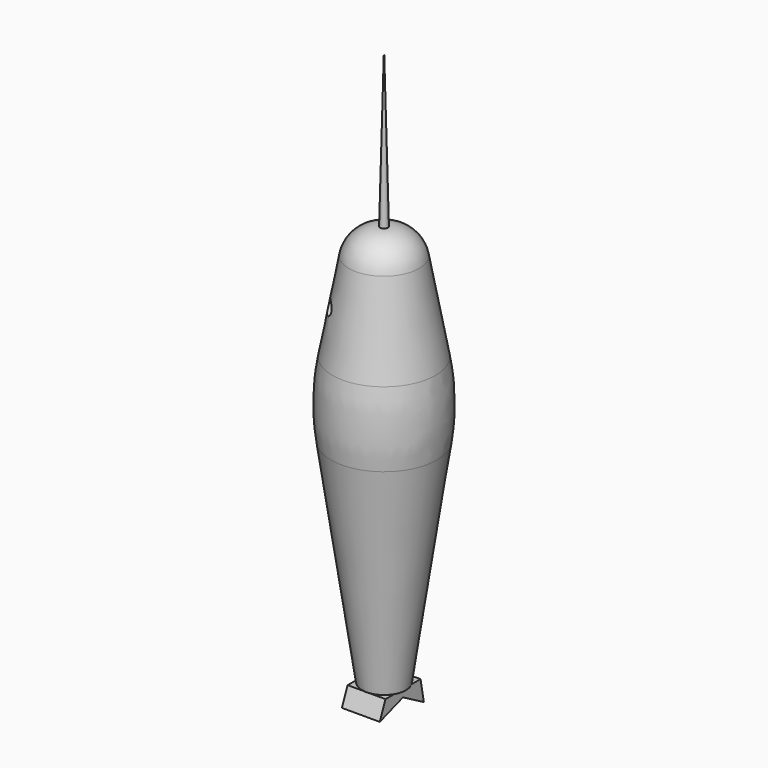
from build123d import *

# Parameters (mm, degrees)
F2_R      = 20.3245328948
F1_R      = 39.0974153035
F4_R      = 21.0995662857
F5_R      = 2.5836298092
F3_FACE_R = 39.0974153035
F10_R     = 14.6545023438
F12_R     = 152.4
F14_DEPTH = 12.7
F15_DEPTH = 12.7
F16_R     = 3.4719949567
F16_R_2   = 4.7718005113
F17_DEPTH = 25.4


with BuildPart() as f3:
    # F2 (on offset) → F3 section 0
    with BuildSketch(Plane.XY.offset(101.6)):
        Circle(F2_R)
    # F1 (on Top) → F3 section 1
    with BuildSketch(Plane.XY):
        Circle(F1_R)
    loft()

    # F4
    f4_edges = [f3.edges().sort_by_distance(p)[0] for p in [
        (-20.324533, 0, 101.6),
    ]]
    fillet(f4_edges, radius=F4_R)

    # F5 (on offset) → F8 section 0
    with BuildSketch(Plane.XY.offset(101.6), mode=Mode.PRIVATE) as f8_s0:
        Circle(F5_R)
    loft([f8_s0.sketch, Vertex(0, 0, 208.026)])

    # F3_face (on face) → F11 section 0
    with BuildSketch(Plane(origin=(0, 0, 0), x_dir=(1, 0, 0), z_dir=(0, 0, -1))):
        Circle(F3_FACE_R)
    # F10 (on offset) → F11 section 1
    with BuildSketch(Plane.XY.offset(-167.64)):
        Circle(F10_R)
    loft()

    # F12
    f12_edges = [f3.edges().sort_by_distance(p)[0] for p in [
        (-39.097415, 0, 0),
    ]]
    fillet(f12_edges, radius=F12_R)

    # F13 (on Right) → F14 (join)
    with BuildSketch(Plane.YZ):
        Polygon((14.7928362712, -167.672470212), (-14.6080739796, -167.5585210323), (-19.3942692131, -179.0681779385), (0, -172.4586635828), (17.5278056413, -182.3729276657), align=None)
    extrude(amount=F14_DEPTH)

    # F13 (on Right) → F15 (join)
    with BuildSketch(Plane.YZ):
        Polygon((14.7928362712, -167.672470212), (-14.6080739796, -167.5585210323), (-19.3942692131, -179.0681779385), (0, -172.4586635828), (17.5278056413, -182.3729276657), align=None)
    extrude(amount=-F15_DEPTH)

    # F16 (on Right) → F17 (cut)
    with BuildSketch(Plane.YZ):
        with Locations((22.7732714266, 55.7852126658)):
            Circle(F16_R)
        with Locations((-19.15024966, 54.7500625253)):
            Circle(F16_R_2)
    extrude(amount=-F17_DEPTH, mode=Mode.SUBTRACT)


solid = f3.part
